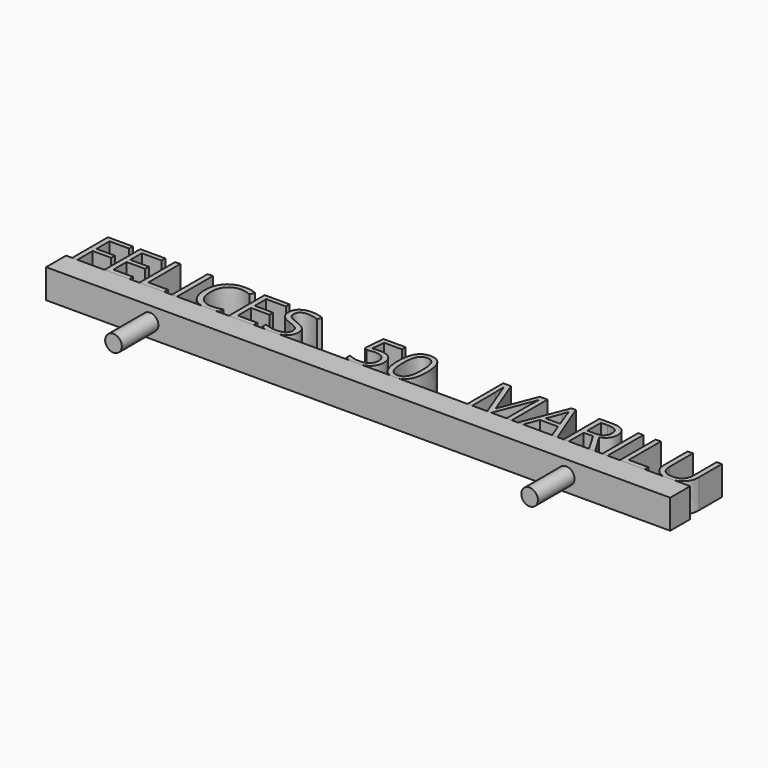
from build123d import *

# Parameters (mm, degrees)
F0_TEXT_SIZE = 15.0571701931
F1_DEPTH     = 7
F2_W         = 150
F2_H         = 6
F3_DEPTH     = 7
F5_DEPTH     = 4
F6_R         = 2
F7_DEPTH     = 11


# Not quite as in the source:
# - Text() gives the source's letters only with a copy of the font that has no kerning and outlines rounded to 1/6400 em; it was checked with that copy


with BuildPart() as f1:
    # F0 (on Top) → F1 (new body)
    with BuildSketch(Plane.XY):
        with Locations((-150, 0)):
            Text('FELICES   50   MARILU', F0_TEXT_SIZE, font='Open Sans', text_align=(TextAlign.LEFT, TextAlign.BOTTOM))
    extrude(amount=F1_DEPTH)


with BuildPart() as f3:
    # F2 (on Top) → F3 (new body)
    with BuildSketch(Plane.XY):
        with Locations((-75, -3)):
            Rectangle(F2_W, F2_H)
    extrude(amount=F3_DEPTH)

    # F4 (on face) → F5 (cut)
    with BuildSketch(Plane(origin=(0, 0, 0), x_dir=(-1, 0, 0), z_dir=(0, 1, 0))):
        with BuildLine():
            ThreePointArc((45.0080148876, 3.25), (44.1241314111, 1.1161165235), (46.2580148876, 2))
            ThreePointArc((46.2580148876, 2), (45.8918983641, 2.8838834765), (45.0080148876, 3.25))
        make_face()
        with BuildLine():
            ThreePointArc((15.8804543316, 3.25), (14.9965708552, 1.1161165235), (17.1304543316, 2))
            ThreePointArc((17.1304543316, 2), (16.7643378081, 2.8838834765), (15.8804543316, 3.25))
        make_face()
        with BuildLine():
            ThreePointArc((90.090110898, 6.5), (88.3223439451, 2.232233047), (92.590110898, 4))
            ThreePointArc((92.590110898, 4), (91.857877851, 5.767766953), (90.090110898, 6.5))
        make_face()
        with BuildLine():
            ThreePointArc((60.1027550697, 6.5), (58.3349881168, 2.232233047), (62.6027550697, 4))
            ThreePointArc((62.6027550697, 4), (61.8705220227, 5.767766953), (60.1027550697, 6.5))
        make_face()
    extrude(amount=-F5_DEPTH, mode=Mode.SUBTRACT)

    # F6 (on face) → F7 (join)
    with BuildSketch(Plane.XZ.offset(6)):
        with BuildLine():
            ThreePointArc((-127, 3.5), (-125, 1.5), (-123, 3.5))
            ThreePointArc((-123, 3.5), (-125, 5.5), (-127, 3.5))
        make_face()
        with Locations((-25, 3.5)):
            Circle(F6_R)
    extrude(amount=F7_DEPTH)


solid = Compound([f1.part, f3.part])
